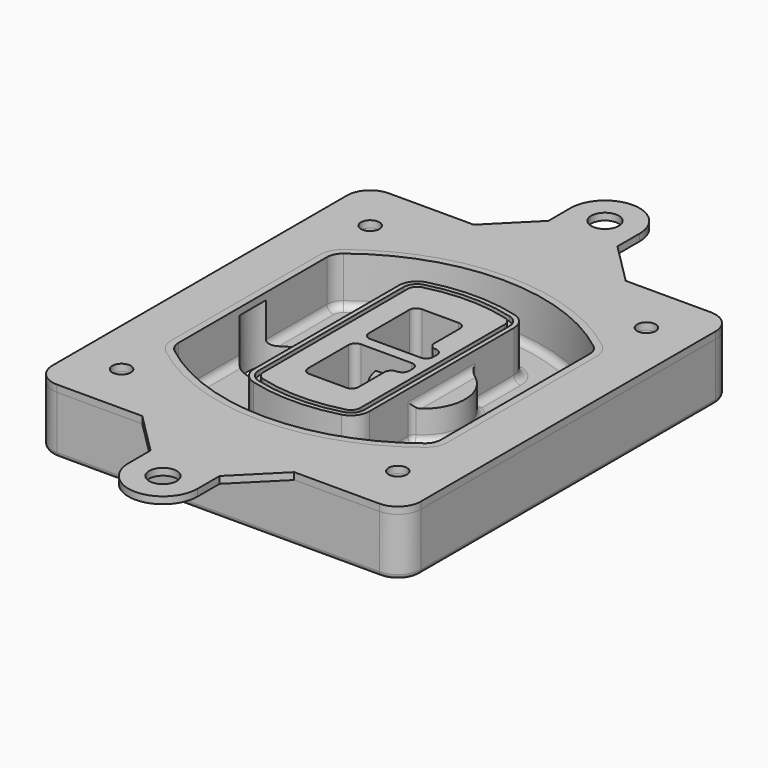
from build123d import *

# Parameters (mm, degrees)
F0_R      = 4
F1_DEPTH  = 25
F2_DEPTH  = 3
F3_DEPTH  = 18
F5_DEPTH  = 21
F6_DEPTH  = 2
F8_DEPTH  = 20
F9_DEPTH  = 16
F10_DEPTH = 25
F7_R      = 6
F7_R_2    = 4
F11_DEPTH = 6
F13_DEPTH = 9
F14_R     = 3
F15_R     = 2
F16_R     = 4
F16_R_2   = 6
F17_DEPTH = 3


# Not quite as in the source:
# - a feature names something its author has since deleted; it is built from what else it names


with BuildPart() as f1:
    # F0 (on Top) → F1 (new body)
    with BuildSketch(Plane.XY):
        with BuildLine():
            ThreePointArc((-80, -80), (-77.0710678119, -87.0710678119), (-70, -90))
            Line((-70, -90), (70, -90))
            ThreePointArc((70, -90), (77.0710678119, -87.0710678119), (80, -80))
            Line((80, -80), (80, 80))
            ThreePointArc((80, 80), (77.0710678119, 87.0710678119), (70, 90))
            Line((70, 90), (-70, 90))
            ThreePointArc((-70, 90), (-77.0710678119, 87.0710678119), (-80, 80))
            Line((-80, 80), (-80, -80))
        make_face()
        with Locations((-60, -67.5)):
            Circle(F0_R, mode=Mode.SUBTRACT)
        with Locations((60, -67.5)):
            Circle(F0_R, mode=Mode.SUBTRACT)
        with Locations((-60, 67.5)):
            Circle(F0_R, mode=Mode.SUBTRACT)
        with BuildLine():
            ThreePointArc((-64, 40.2934422872), (-62.5820384798, 46.4328484224), (-58.6153846154, 51.3286200352))
            ThreePointArc((-58.6153846154, 51.3286200352), (0, 71.5), (58.6153846154, 51.3286200352))
            ThreePointArc((58.6153846154, 51.3286200352), (62.5820384798, 46.4328484224), (64, 40.2934422872))
            Line((64, 40.2934422872), (64, -40.2934422872))
            ThreePointArc((64, -40.2934422872), (62.5820384798, -46.4328484224), (58.6153846154, -51.3286200352))
            ThreePointArc((58.6153846154, -51.3286200352), (0, -71.5), (-58.6153846154, -51.3286200352))
            ThreePointArc((-58.6153846154, -51.3286200352), (-62.5820384798, -46.4328484224), (-64, -40.2934422872))
            Line((-64, -40.2934422872), (-64, 40.2934422872))
        make_face(mode=Mode.SUBTRACT)
        with Locations((60, 67.5)):
            Circle(F0_R, mode=Mode.SUBTRACT)
        with BuildLine():
            ThreePointArc((58.6153846154, 51.3286200352), (0, 71.5), (-58.6153846154, 51.3286200352))
            ThreePointArc((-58.6153846154, 51.3286200352), (-62.5820384798, 46.4328484224), (-64, 40.2934422872))
            Line((-64, 40.2934422872), (-64, -40.2934422872))
            ThreePointArc((-64, -40.2934422872), (-62.5820384798, -46.4328484224), (-58.6153846154, -51.3286200352))
            ThreePointArc((-58.6153846154, -51.3286200352), (0, -71.5), (58.6153846154, -51.3286200352))
            ThreePointArc((58.6153846154, -51.3286200352), (62.5820384798, -46.4328484224), (64, -40.2934422872))
            Line((64, -40.2934422872), (64, 40.2934422872))
            ThreePointArc((64, 40.2934422872), (62.5820384798, 46.4328484224), (58.6153846154, 51.3286200352))
        make_face()
        with BuildLine():
            Line((-60, -40.2934422872), (-60, 40.2934422872))
            ThreePointArc((-60, 40.2934422872), (-58.9871703427, 44.6787323838), (-56.1538461538, 48.1757121072))
            ThreePointArc((-56.1538461538, 48.1757121072), (0, 67.5), (56.1538461538, 48.1757121072))
            ThreePointArc((56.1538461538, 48.1757121072), (58.9871703427, 44.6787323838), (60, 40.2934422872))
            Line((60, 40.2934422872), (60, -40.2934422872))
            ThreePointArc((60, -40.2934422872), (58.9871703427, -44.6787323838), (56.1538461538, -48.1757121072))
            ThreePointArc((56.1538461538, -48.1757121072), (0, -67.5), (-56.1538461538, -48.1757121072))
            ThreePointArc((-56.1538461538, -48.1757121072), (-58.9871703427, -44.6787323838), (-60, -40.2934422872))
        make_face(mode=Mode.SUBTRACT)
        with BuildLine():
            ThreePointArc((-56.1538461538, 48.1757121072), (-58.9871703427, 44.6787323838), (-60, 40.2934422872))
            Line((-60, 40.2934422872), (-60, -40.2934422872))
            ThreePointArc((-60, -40.2934422872), (-58.9871703427, -44.6787323838), (-56.1538461538, -48.1757121072))
            ThreePointArc((-56.1538461538, -48.1757121072), (0, -67.5), (56.1538461538, -48.1757121072))
            ThreePointArc((56.1538461538, -48.1757121072), (58.9871703427, -44.6787323838), (60, -40.2934422872))
            Line((60, -40.2934422872), (60, 40.2934422872))
            ThreePointArc((60, 40.2934422872), (58.9871703427, 44.6787323838), (56.1538461538, 48.1757121072))
            ThreePointArc((56.1538461538, 48.1757121072), (0, 67.5), (-56.1538461538, 48.1757121072))
        make_face()
        with BuildLine():
            ThreePointArc((54.3076923077, 45.8110311612), (56.2910192399, 43.3631453548), (57, 40.2934422872))
            Line((57, 40.2934422872), (57, -40.2934422872))
            ThreePointArc((57, -40.2934422872), (56.2910192399, -43.3631453548), (54.3076923077, -45.8110311612))
            ThreePointArc((54.3076923077, -45.8110311612), (0, -64.5), (-54.3076923077, -45.8110311612))
            ThreePointArc((-54.3076923077, -45.8110311612), (-56.2910192399, -43.3631453548), (-57, -40.2934422872))
            Line((-57, -40.2934422872), (-57, 40.2934422872))
            ThreePointArc((-57, 40.2934422872), (-56.2910192399, 43.3631453548), (-54.3076923077, 45.8110311612))
            ThreePointArc((-54.3076923077, 45.8110311612), (0, 64.5), (54.3076923077, 45.8110311612))
        make_face(mode=Mode.SUBTRACT)
        with BuildLine():
            Line((57, -40.2934422872), (57, 40.2934422872))
            ThreePointArc((57, 40.2934422872), (56.2910192399, 43.3631453548), (54.3076923077, 45.8110311612))
            ThreePointArc((54.3076923077, 45.8110311612), (0, 64.5), (-54.3076923077, 45.8110311612))
            ThreePointArc((-54.3076923077, 45.8110311612), (-56.2910192399, 43.3631453548), (-57, 40.2934422872))
            Line((-57, 40.2934422872), (-57, -40.2934422872))
            ThreePointArc((-57, -40.2934422872), (-56.2910192399, -43.3631453548), (-54.3076923077, -45.8110311612))
            ThreePointArc((-54.3076923077, -45.8110311612), (0, -64.5), (54.3076923077, -45.8110311612))
            ThreePointArc((54.3076923077, -45.8110311612), (56.2910192399, -43.3631453548), (57, -40.2934422872))
        make_face()
    extrude(amount=-F1_DEPTH)

    # F0 (on Top) → F2 (join)
    with BuildSketch(Plane.XY):
        with BuildLine():
            ThreePointArc((-56.1538461538, 48.1757121072), (-58.9871703427, 44.6787323838), (-60, 40.2934422872))
            Line((-60, 40.2934422872), (-60, -40.2934422872))
            ThreePointArc((-60, -40.2934422872), (-58.9871703427, -44.6787323838), (-56.1538461538, -48.1757121072))
            ThreePointArc((-56.1538461538, -48.1757121072), (0, -67.5), (56.1538461538, -48.1757121072))
            ThreePointArc((56.1538461538, -48.1757121072), (58.9871703427, -44.6787323838), (60, -40.2934422872))
            Line((60, -40.2934422872), (60, 40.2934422872))
            ThreePointArc((60, 40.2934422872), (58.9871703427, 44.6787323838), (56.1538461538, 48.1757121072))
            ThreePointArc((56.1538461538, 48.1757121072), (0, 67.5), (-56.1538461538, 48.1757121072))
        make_face()
        with BuildLine():
            ThreePointArc((54.3076923077, 45.8110311612), (56.2910192399, 43.3631453548), (57, 40.2934422872))
            Line((57, 40.2934422872), (57, -40.2934422872))
            ThreePointArc((57, -40.2934422872), (56.2910192399, -43.3631453548), (54.3076923077, -45.8110311612))
            ThreePointArc((54.3076923077, -45.8110311612), (0, -64.5), (-54.3076923077, -45.8110311612))
            ThreePointArc((-54.3076923077, -45.8110311612), (-56.2910192399, -43.3631453548), (-57, -40.2934422872))
            Line((-57, -40.2934422872), (-57, 40.2934422872))
            ThreePointArc((-57, 40.2934422872), (-56.2910192399, 43.3631453548), (-54.3076923077, 45.8110311612))
            ThreePointArc((-54.3076923077, 45.8110311612), (0, 64.5), (54.3076923077, 45.8110311612))
        make_face(mode=Mode.SUBTRACT)
    extrude(amount=F2_DEPTH)

    # F0 (on Top) → F3 (cut)
    with BuildSketch(Plane.XY):
        with BuildLine():
            Line((57, -40.2934422872), (57, 40.2934422872))
            ThreePointArc((57, 40.2934422872), (56.2910192399, 43.3631453548), (54.3076923077, 45.8110311612))
            ThreePointArc((54.3076923077, 45.8110311612), (0, 64.5), (-54.3076923077, 45.8110311612))
            ThreePointArc((-54.3076923077, 45.8110311612), (-56.2910192399, 43.3631453548), (-57, 40.2934422872))
            Line((-57, 40.2934422872), (-57, -40.2934422872))
            ThreePointArc((-57, -40.2934422872), (-56.2910192399, -43.3631453548), (-54.3076923077, -45.8110311612))
            ThreePointArc((-54.3076923077, -45.8110311612), (0, -64.5), (54.3076923077, -45.8110311612))
            ThreePointArc((54.3076923077, -45.8110311612), (56.2910192399, -43.3631453548), (57, -40.2934422872))
        make_face()
    extrude(amount=-F3_DEPTH, mode=Mode.SUBTRACT)

    # F4 (on face) → F5 (join, through all)
    with BuildSketch(Plane.XY.offset(3)):
        with BuildLine():
            ThreePointArc((-25, -39.2465276821), (-23.3511545998, -44.1109737193), (-19.0842911877, -46.9702398883))
            ThreePointArc((-19.0842911877, -46.9702398883), (0, -49.5), (19.0842911877, -46.9702398883))
            ThreePointArc((19.0842911877, -46.9702398883), (23.3511545998, -44.1109737193), (25, -39.2465276821))
            Line((25, -39.2465276821), (25, 39.2465276821))
            ThreePointArc((25, 39.2465276821), (23.3511545998, 44.1109737193), (19.0842911877, 46.9702398883))
            ThreePointArc((19.0842911877, 46.9702398883), (0, 49.5), (-19.0842911877, 46.9702398883))
            ThreePointArc((-19.0842911877, 46.9702398883), (-23.3511545998, 44.1109737193), (-25, 39.2465276821))
            Line((-25, 39.2465276821), (-25, -39.2465276821))
        make_face()
        with BuildLine():
            ThreePointArc((18.5632183908, 45.0393118368), (21.7633659499, 42.89486221), (23, 39.2465276821))
            Line((23, 39.2465276821), (23, -39.2465276821))
            ThreePointArc((23, -39.2465276821), (21.7633659499, -42.89486221), (18.5632183908, -45.0393118368))
            ThreePointArc((18.5632183908, -45.0393118368), (0, -47.5), (-18.5632183908, -45.0393118368))
            ThreePointArc((-18.5632183908, -45.0393118368), (-21.7633659499, -42.89486221), (-23, -39.2465276821))
            Line((-23, -39.2465276821), (-23, 39.2465276821))
            ThreePointArc((-23, 39.2465276821), (-21.7633659499, 42.89486221), (-18.5632183908, 45.0393118368))
            ThreePointArc((-18.5632183908, 45.0393118368), (0, 47.5), (18.5632183908, 45.0393118368))
        make_face(mode=Mode.SUBTRACT)
        with BuildLine():
            Line((23, -39.2465276821), (23, 39.2465276821))
            ThreePointArc((23, 39.2465276821), (21.7633659499, 42.89486221), (18.5632183908, 45.0393118368))
            ThreePointArc((18.5632183908, 45.0393118368), (0, 47.5), (-18.5632183908, 45.0393118368))
            ThreePointArc((-18.5632183908, 45.0393118368), (-21.7633659499, 42.89486221), (-23, 39.2465276821))
            Line((-23, 39.2465276821), (-23, -39.2465276821))
            ThreePointArc((-23, -39.2465276821), (-21.7633659499, -42.89486221), (-18.5632183908, -45.0393118368))
            ThreePointArc((-18.5632183908, -45.0393118368), (0, -47.5), (18.5632183908, -45.0393118368))
            ThreePointArc((18.5632183908, -45.0393118368), (21.7633659499, -42.89486221), (23, -39.2465276821))
        make_face()
        with BuildLine():
            ThreePointArc((18.0421455939, 43.1083837852), (20.1755772999, 41.6787507007), (21, 39.2465276821))
            Line((21, 39.2465276821), (21, -39.2465276821))
            ThreePointArc((21, -39.2465276821), (20.1755772999, -41.6787507007), (18.0421455939, -43.1083837852))
            ThreePointArc((18.0421455939, -43.1083837852), (0, -45.5), (-18.0421455939, -43.1083837852))
            ThreePointArc((-18.0421455939, -43.1083837852), (-20.1755772999, -41.6787507007), (-21, -39.2465276821))
            Line((-21, -39.2465276821), (-21, 39.2465276821))
            ThreePointArc((-21, 39.2465276821), (-20.1755772999, 41.6787507007), (-18.0421455939, 43.1083837852))
            ThreePointArc((-18.0421455939, 43.1083837852), (0, 45.5), (18.0421455939, 43.1083837852))
        make_face(mode=Mode.SUBTRACT)
        with BuildLine():
            Line((21, -39.2465276821), (21, 39.2465276821))
            ThreePointArc((21, 39.2465276821), (20.1755772999, 41.6787507007), (18.0421455939, 43.1083837852))
            ThreePointArc((18.0421455939, 43.1083837852), (0, 45.5), (-18.0421455939, 43.1083837852))
            ThreePointArc((-18.0421455939, 43.1083837852), (-20.1755772999, 41.6787507007), (-21, 39.2465276821))
            Line((-21, 39.2465276821), (-21, -39.2465276821))
            ThreePointArc((-21, -39.2465276821), (-20.1755772999, -41.6787507007), (-18.0421455939, -43.1083837852))
            ThreePointArc((-18.0421455939, -43.1083837852), (0, -45.5), (18.0421455939, -43.1083837852))
            ThreePointArc((18.0421455939, -43.1083837852), (20.1755772999, -41.6787507007), (21, -39.2465276821))
        make_face()
        with BuildLine():
            Line((-8, -2.5), (14, -2.5))
            ThreePointArc((14, -2.5), (16.1213203436, -3.3786796564), (17, -5.5))
            Line((17, -5.5), (17, -7.5))
            ThreePointArc((17, -7.5), (16.1213203436, -9.6213203436), (14, -10.5))
            ThreePointArc((14, -10.5), (11.8786796564, -11.3786796564), (11, -13.5))
            Line((11, -13.5), (11, -27.5))
            ThreePointArc((11, -27.5), (10.1213203436, -29.6213203436), (8, -30.5))
            Line((8, -30.5), (-8, -30.5))
            ThreePointArc((-8, -30.5), (-10.1213203436, -29.6213203436), (-11, -27.5))
            Line((-11, -27.5), (-11, -5.5))
            ThreePointArc((-11, -5.5), (-10.1213203436, -3.3786796564), (-8, -2.5))
        make_face(mode=Mode.SUBTRACT)
        with BuildLine():
            ThreePointArc((-8, 2.5), (-10.1213203436, 3.3786796564), (-11, 5.5))
            Line((-11, 5.5), (-11, 27.5))
            ThreePointArc((-11, 27.5), (-10.1213203436, 29.6213203436), (-8, 30.5))
            Line((-8, 30.5), (8, 30.5))
            ThreePointArc((8, 30.5), (10.1213203436, 29.6213203436), (11, 27.5))
            Line((11, 27.5), (11, 13.5))
            ThreePointArc((11, 13.5), (11.8786796564, 11.3786796564), (14, 10.5))
            ThreePointArc((14, 10.5), (16.1213203436, 9.6213203436), (17, 7.5))
            Line((17, 7.5), (17, 5.5))
            ThreePointArc((17, 5.5), (16.1213203436, 3.3786796564), (14, 2.5))
            Line((14, 2.5), (-8, 2.5))
        make_face(mode=Mode.SUBTRACT)
    extrude(amount=-F5_DEPTH)

    # F4 (on face) → F6 (cut)
    with BuildSketch(Plane.XY.offset(3)):
        with BuildLine():
            Line((23, -39.2465276821), (23, 39.2465276821))
            ThreePointArc((23, 39.2465276821), (21.7633659499, 42.89486221), (18.5632183908, 45.0393118368))
            ThreePointArc((18.5632183908, 45.0393118368), (0, 47.5), (-18.5632183908, 45.0393118368))
            ThreePointArc((-18.5632183908, 45.0393118368), (-21.7633659499, 42.89486221), (-23, 39.2465276821))
            Line((-23, 39.2465276821), (-23, -39.2465276821))
            ThreePointArc((-23, -39.2465276821), (-21.7633659499, -42.89486221), (-18.5632183908, -45.0393118368))
            ThreePointArc((-18.5632183908, -45.0393118368), (0, -47.5), (18.5632183908, -45.0393118368))
            ThreePointArc((18.5632183908, -45.0393118368), (21.7633659499, -42.89486221), (23, -39.2465276821))
        make_face()
        with BuildLine():
            ThreePointArc((18.0421455939, 43.1083837852), (20.1755772999, 41.6787507007), (21, 39.2465276821))
            Line((21, 39.2465276821), (21, -39.2465276821))
            ThreePointArc((21, -39.2465276821), (20.1755772999, -41.6787507007), (18.0421455939, -43.1083837852))
            ThreePointArc((18.0421455939, -43.1083837852), (0, -45.5), (-18.0421455939, -43.1083837852))
            ThreePointArc((-18.0421455939, -43.1083837852), (-20.1755772999, -41.6787507007), (-21, -39.2465276821))
            Line((-21, -39.2465276821), (-21, 39.2465276821))
            ThreePointArc((-21, 39.2465276821), (-20.1755772999, 41.6787507007), (-18.0421455939, 43.1083837852))
            ThreePointArc((-18.0421455939, 43.1083837852), (0, 45.5), (18.0421455939, 43.1083837852))
        make_face(mode=Mode.SUBTRACT)
    extrude(amount=-F6_DEPTH, mode=Mode.SUBTRACT)

    # F7 (on face) → F8 (join)
    with BuildSketch(Plane(origin=(0, 0, -25), x_dir=(1, 0, 0), z_dir=(0, 0, -1))):
        with BuildLine():
            ThreePointArc((3.28842436, 0), (16.7567035675, 13.4682792075), (30.224982775, 0))
            Line((30.224982775, 0), (35.224982775, 0))
            ThreePointArc((35.224982775, 0), (16.7567035675, 18.4682792075), (-1.71157564, 0))
            Line((-1.71157564, 0), (3.28842436, 0))
        make_face()
        with BuildLine():
            Line((3.28842436, 0), (30.224982775, 0))
            ThreePointArc((30.224982775, 0), (16.7567035675, 13.4682792075), (3.28842436, 0))
        make_face()
        with BuildLine():
            ThreePointArc((3.28842436, 0), (16.7567035675, -13.4682792075), (30.224982775, 0))
            Line((30.224982775, 0), (3.28842436, 0))
        make_face()
        with BuildLine():
            Line((35.224982775, 0), (30.224982775, 0))
            ThreePointArc((30.224982775, 0), (16.7567035675, -13.4682792075), (3.28842436, 0))
            Line((3.28842436, 0), (-1.71157564, 0))
            ThreePointArc((-1.71157564, 0), (16.7567035675, -18.4682792075), (35.224982775, 0))
        make_face()
    extrude(amount=-F8_DEPTH)

    # F7 (on face) → F9 (cut)
    with BuildSketch(Plane(origin=(0, 0, -25), x_dir=(1, 0, 0), z_dir=(0, 0, -1))):
        with BuildLine():
            Line((3.28842436, 0), (30.224982775, 0))
            ThreePointArc((30.224982775, 0), (16.7567035675, 13.4682792075), (3.28842436, 0))
        make_face()
        with BuildLine():
            ThreePointArc((3.28842436, 0), (16.7567035675, -13.4682792075), (30.224982775, 0))
            Line((30.224982775, 0), (3.28842436, 0))
        make_face()
    extrude(amount=-F9_DEPTH, mode=Mode.SUBTRACT)

    # F7 (on face) → F10 (cut)
    with BuildSketch(Plane(origin=(0, 0, -25), x_dir=(1, 0, 0), z_dir=(0, 0, -1))):
        with BuildLine():
            Line((-59.0318229325, 0), (-32.0952645175, 0))
            ThreePointArc((-32.0952645175, 0), (-45.563543725, 13.4682792075), (-59.0318229325, 0))
        make_face()
        with BuildLine():
            ThreePointArc((-59.0318229325, 0), (-45.563543725, -13.4682792075), (-32.0952645175, 0))
            Line((-32.0952645175, 0), (-59.0318229325, 0))
        make_face()
    extrude(amount=-F10_DEPTH, mode=Mode.SUBTRACT)

    # F7 (on face) → F11 (cut)
    with BuildSketch(Plane(origin=(0, 0, -25), x_dir=(1, 0, 0), z_dir=(0, 0, -1))):
        with Locations((60, -67.5)):
            Circle(F7_R)
        with Locations((60, -67.5)):
            Circle(F7_R_2, mode=Mode.SUBTRACT)
        with Locations((-60, -67.5)):
            Circle(F7_R)
        with Locations((-60, -67.5)):
            Circle(F7_R_2, mode=Mode.SUBTRACT)
        with Locations((-60, 67.5)):
            Circle(F7_R)
        with Locations((-60, 67.5)):
            Circle(F7_R_2, mode=Mode.SUBTRACT)
        with Locations((60, 67.5)):
            Circle(F7_R)
        with Locations((60, 67.5)):
            Circle(F7_R_2, mode=Mode.SUBTRACT)
    extrude(amount=-F11_DEPTH, mode=Mode.SUBTRACT)

    # F12 (on face) → F13 (cut, through all)
    with BuildSketch(Plane(origin=(0, 0, -9), x_dir=(1, 0, 0), z_dir=(0, 0, -1))):
        with BuildLine():
            Line((11, 13.5), (11, 17.5481537753))
            ThreePointArc((11, 17.5481537753), (2.5696536419, 11.8239143813), (-1.5415842455, 2.5))
            Line((-1.5415842455, 2.5), (3.5224848595, 2.5))
            ThreePointArc((3.5224848595, 2.5), (6.1857188154, 8.3455872281), (11.2536447004, 12.2927168648))
            ThreePointArc((11.2536447004, 12.2927168648), (11.0640958889, 12.8831798879), (11, 13.5))
        make_face()
        with BuildLine():
            ThreePointArc((11.2536447004, -12.2927168648), (6.1857188154, -8.3455872281), (3.5224848595, -2.5))
            Line((3.5224848595, -2.5), (-1.5415842455, -2.5))
            ThreePointArc((-1.5415842455, -2.5), (2.5696536419, -11.8239143813), (11, -17.5481537753))
            Line((11, -17.5481537753), (11, -13.5))
            ThreePointArc((11, -13.5), (11.0640958889, -12.8831798879), (11.2536447004, -12.2927168648))
        make_face()
        with BuildLine():
            ThreePointArc((11.2536447004, 12.2927168648), (6.1857188154, 8.3455872281), (3.5224848595, 2.5))
            Line((3.5224848595, 2.5), (14, 2.5))
            ThreePointArc((14, 2.5), (16.1213203436, 3.3786796564), (17, 5.5))
            Line((17, 5.5), (17, 7.5))
            ThreePointArc((17, 7.5), (16.1213203436, 9.6213203436), (14, 10.5))
            ThreePointArc((14, 10.5), (12.3601599782, 10.9878446101), (11.2536447004, 12.2927168648))
        make_face()
        with BuildLine():
            Line((14, -2.5), (3.5224848595, -2.5))
            ThreePointArc((3.5224848595, -2.5), (6.1857188154, -8.3455872281), (11.2536447004, -12.2927168648))
            ThreePointArc((11.2536447004, -12.2927168648), (12.3601599782, -10.9878446101), (14, -10.5))
            ThreePointArc((14, -10.5), (16.1213203436, -9.6213203436), (17, -7.5))
            Line((17, -7.5), (17, -5.5))
            ThreePointArc((17, -5.5), (16.1213203436, -3.3786796564), (14, -2.5))
        make_face()
    extrude(amount=F13_DEPTH, mode=Mode.SUBTRACT)

    # F14
    f14_edges = [f1.edges().sort_by_distance(p)[0] for p in [
        (-57, -23.703476, -18),
        (-57, 23.703476, -18),
        (25, 0, -5),
        (25, 16.526506, -11.5),
        (25, -16.526506, -11.5),
        (25, -27.886517, -18),
        (35.224983, 0, -18),
    ]]
    fillet(f14_edges, radius=F14_R)

    # F15
    f15_edges = [f1.edges().sort_by_distance(p)[0] for p in [
        (0, -90, -25),
    ]]
    fillet(f15_edges, radius=F15_R)


with BuildPart() as f17:
    # F16 (on face) → F17 (new body, through all)
    with BuildSketch(Plane.XY):
        with BuildLine():
            Line((-33, 90), (-70, 90))
            ThreePointArc((-70, 90), (-77.0710678119, 87.0710678119), (-80, 80))
            Line((-80, 80), (-80, -80))
            ThreePointArc((-80, -80), (-77.0710678119, -87.0710678119), (-70, -90))
            Line((-70, -90), (-33, -90))
            Line((-33, -90), (33, -90))
            Line((33, -90), (70, -90))
            ThreePointArc((70, -90), (77.0710678119, -87.0710678119), (80, -80))
            Line((80, -80), (80, 80))
            ThreePointArc((80, 80), (77.0710678119, 87.0710678119), (70, 90))
            Line((70, 90), (33, 90))
            Line((33, 90), (-33, 90))
        make_face()
        with Locations((-60, -67.5)):
            Circle(F16_R, mode=Mode.SUBTRACT)
        with Locations((60, -67.5)):
            Circle(F16_R, mode=Mode.SUBTRACT)
        with Locations((-60, 67.5)):
            Circle(F16_R, mode=Mode.SUBTRACT)
        with BuildLine():
            ThreePointArc((-60, 40.2934422872), (-58.9871703427, 44.6787323838), (-56.1538461538, 48.1757121072))
            ThreePointArc((-56.1538461538, 48.1757121072), (0, 67.5), (56.1538461538, 48.1757121072))
            ThreePointArc((56.1538461538, 48.1757121072), (58.9871703427, 44.6787323838), (60, 40.2934422872))
            Line((60, 40.2934422872), (60, -40.2934422872))
            ThreePointArc((60, -40.2934422872), (58.9871703427, -44.6787323838), (56.1538461538, -48.1757121072))
            ThreePointArc((56.1538461538, -48.1757121072), (0, -67.5), (-56.1538461538, -48.1757121072))
            ThreePointArc((-56.1538461538, -48.1757121072), (-58.9871703427, -44.6787323838), (-60, -40.2934422872))
            Line((-60, -40.2934422872), (-60, 40.2934422872))
        make_face(mode=Mode.SUBTRACT)
        with Locations((60, 67.5)):
            Circle(F16_R, mode=Mode.SUBTRACT)
        with BuildLine():
            Line((-15, 108), (-33, 90))
            Line((-33, 90), (33, 90))
            Line((33, 90), (15, 108))
            Line((15, 108), (15, 120))
            ThreePointArc((15, 120), (0, 135), (-15, 120))
            Line((-15, 120), (-15, 108))
        make_face()
        with Locations((0, 120)):
            Circle(F16_R_2, mode=Mode.SUBTRACT)
        with BuildLine():
            Line((33, -90), (-33, -90))
            Line((-33, -90), (-15, -108))
            Line((-15, -108), (-15, -120))
            ThreePointArc((-15, -120), (0, -135), (15, -120))
            Line((15, -120), (15, -108))
            Line((15, -108), (33, -90))
        make_face()
        with Locations((0, -120)):
            Circle(F16_R_2, mode=Mode.SUBTRACT)
    extrude(amount=F17_DEPTH)


solid = Compound([f1.part, f17.part])
